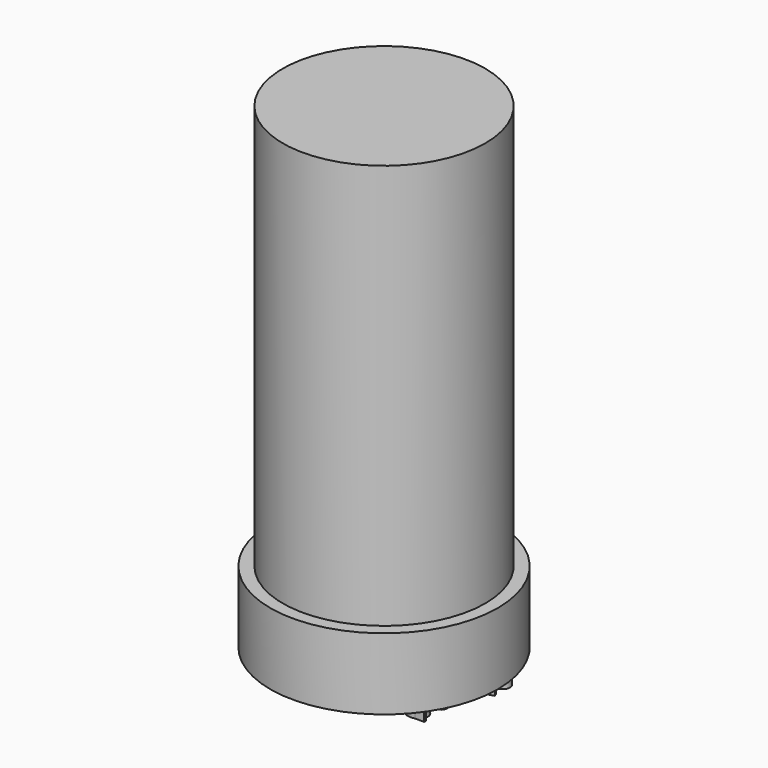
from build123d import *

# Parameters (mm, degrees)
F0_R         = 10.795
F1_DEPTH     = 50.8
F0_R_2       = 12.1285
F2_DEPTH     = 7.62
F3_TEXT_SIZE = 5.3033048831
F4_DEPTH     = 1.27


# Not quite as in the source:
# - Text() gives the source's letters only with a copy of the font that has no kerning and outlines rounded to 1/6400 em; it was checked with that copy


with BuildPart() as f1:
    # F0 (on Top) → F1 (new body)
    with BuildSketch(Plane.XY):
        Circle(F0_R)
    extrude(amount=F1_DEPTH)

    # F0 (on Top) → F2 (join)
    with BuildSketch(Plane.XY):
        Circle(F0_R_2)
        Circle(F0_R, mode=Mode.SUBTRACT)
    extrude(amount=F2_DEPTH)

    # F3 (on face) → F4 (join)
    with BuildSketch(Plane(origin=(0, 0, 0), x_dir=(1, 0, 0), z_dir=(0, 0, -1))):
        with Locations((-9.5300138296, 3.6835768061)):
            Text('He-Xing', F3_TEXT_SIZE, font='Open Sans', text_align=(TextAlign.LEFT, TextAlign.BOTTOM))
        with Locations((-9.5300138296, -3.5289178349)):
            Text('Gardens', F3_TEXT_SIZE, font='Open Sans', text_align=(TextAlign.LEFT, TextAlign.BOTTOM))
    extrude(amount=F4_DEPTH)


solid = f1.part
